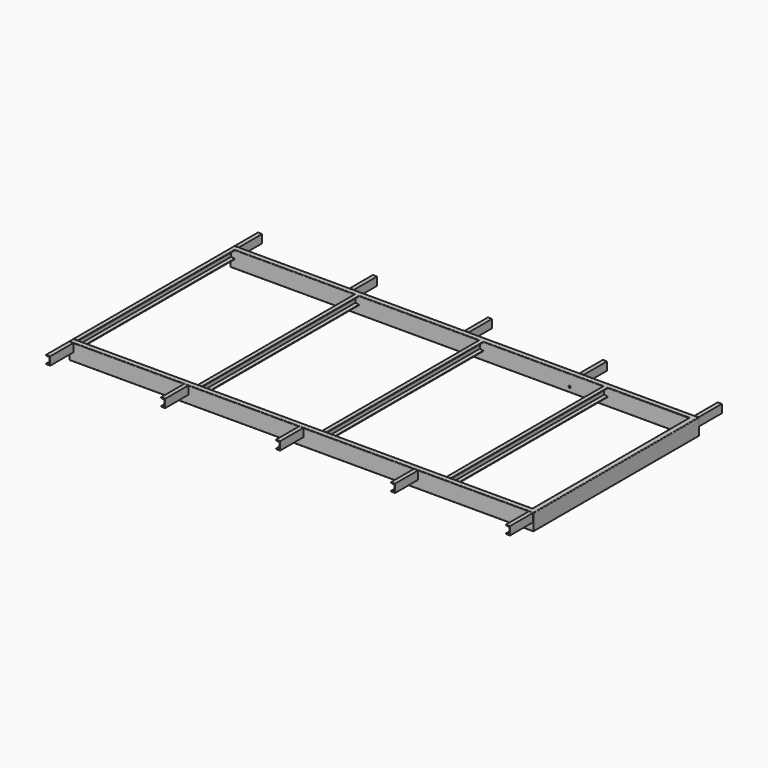
from build123d import *

# Parameters (mm, degrees)
F1_W      = 31.75
F1_H      = 133.35
F5_W      = 38.1
F5_H      = 5
F6_DEPTH  = 266.7
F7_W      = 38.1
F7_H      = 5
F8_DEPTH  = 266.7
F9_R      = 9.525
F10_DEPTH = 2640


with BuildPart() as f2:
    # F2: sweep along a path in F0
    with BuildLine(Plane.XY) as f2_path:
        Line((0, 0), (4221.5954545455, 0))
        Line((4221.5954545455, 0), (4221.5954545455, 1803.4))
        Line((4221.5954545455, 1803.4), (0, 1803.4))
    # F1 (on Right) → F2 (sweep)
    with BuildSketch(Plane.YZ):
        with BuildLine():
            ThreePointArc((0, -5), (-1.4644660941, -1.4644660941), (-5, 0))
            Line((-5, 0), (-45.8, 0))
            ThreePointArc((-45.8, 0), (-49.3355339059, -1.4644660941), (-50.8, -5))
            Line((-50.8, -5), (-50.8, -147.4))
            ThreePointArc((-50.8, -147.4), (-49.3355339059, -150.9355339059), (-45.8, -152.4))
            Line((-45.8, -152.4), (-5, -152.4))
            ThreePointArc((-5, -152.4), (-1.4644660941, -150.9355339059), (0, -147.4))
            Line((0, -147.4), (0, -5))
        make_face()
        with Locations((-25.4, -76.2)):
            Rectangle(F1_W, F1_H, mode=Mode.SUBTRACT)
    sweep(path=f2_path.line, transition=Transition.RIGHT)

    # F3 (on face) → F4 (join, up to the next surface of F2)
    with BuildSketch(Plane(origin=(0, 0, 0), x_dir=(-1, 0, 0), z_dir=(0, 1, 0))):
        Polygon((0, 0), (-38.1, 0), (-38.1, -5.08), (-6.35, -10), (-6.35, -66.2), (-38.1, -71.12), (-38.1, -76.2), (0, -76.2), align=None)
        Polygon((-1150.9375, -10), (-1150.9375, -66.2), (-1182.6875, -71.12), (-1182.6875, -76.2), (-1144.5875, -76.2), (-1144.5875, 0), (-1182.6875, 0), (-1182.6875, -5.08), align=None)
        Polygon((-2295.525, -10), (-2295.525, -66.2), (-2327.275, -71.12), (-2327.275, -76.2), (-2289.175, -76.2), (-2289.175, 0), (-2327.275, 0), (-2327.275, -5.08), align=None)
        Polygon((-3440.1125, -10), (-3440.1125, -66.2), (-3471.8625, -71.12), (-3471.8625, -76.2), (-3433.7625, -76.2), (-3433.7625, 0), (-3471.8625, 0), (-3471.8625, -5.08), align=None)
    extrude(until=Until.NEXT)

    # F5 (on face) → F6 (join)
    with BuildSketch(Plane.XZ.offset(50.8)):
        Polygon((38.1, -5), (0, -5), (0, -5.08), (31.75, -10), (31.75, -66.2), (0, -71.12), (0, -76.2), (38.1, -76.2), align=None)
        Polygon((1096.01, -5), (1057.91, -5), (1057.91, -5.08), (1089.66, -10), (1089.66, -66.2), (1057.91, -71.12), (1057.91, -76.2), (1096.01, -76.2), align=None)
        Polygon((2153.92, -5), (2115.82, -5), (2115.82, -5.08), (2147.57, -10), (2147.57, -66.2), (2115.82, -71.12), (2115.82, -76.2), (2153.92, -76.2), align=None)
        Polygon((3211.83, -5), (3173.73, -5), (3173.73, -5.08), (3205.48, -10), (3205.48, -66.2), (3173.73, -71.12), (3173.73, -76.2), (3211.83, -76.2), align=None)
        Polygon((4269.74, -76.2), (4269.74, -5), (4231.64, -5), (4231.64, -5.08), (4263.39, -10), (4263.39, -66.2), (4231.64, -71.12), (4231.64, -76.2), align=None)
        with Locations((4250.69, -2.5)):
            Rectangle(F5_W, F5_H)
        with Locations((3192.78, -2.5)):
            Rectangle(F5_W, F5_H)
        with Locations((2134.87, -2.5)):
            Rectangle(F5_W, F5_H)
        with Locations((1076.96, -2.5)):
            Rectangle(F5_W, F5_H)
        with Locations((19.05, -2.5)):
            Rectangle(F5_W, F5_H)
    extrude(amount=F6_DEPTH)

    # F7 (on face) → F8 (join)
    with BuildSketch(Plane(origin=(0, 1854.2, 0), x_dir=(-1, 0, 0), z_dir=(0, 1, 0))):
        Polygon((0, -5), (-38.1, -5), (-38.1, -76.2), (0, -76.2), (0, -71.12), (-31.75, -66.2), (-31.75, -10), (0, -5.08), align=None)
        with Locations((-19.05, -2.5)):
            Rectangle(F7_W, F7_H)
        with Locations((-1076.96, -2.5)):
            Rectangle(F7_W, F7_H)
        Polygon((-1057.91, -5.08), (-1057.91, -5), (-1096.01, -5), (-1096.01, -76.2), (-1057.91, -76.2), (-1057.91, -71.12), (-1089.66, -66.2), (-1089.66, -10), align=None)
        Polygon((-2115.82, -5.08), (-2115.82, -5), (-2153.92, -5), (-2153.92, -76.2), (-2115.82, -76.2), (-2115.82, -71.12), (-2147.57, -66.2), (-2147.57, -10), align=None)
        with Locations((-2134.87, -2.5)):
            Rectangle(F7_W, F7_H)
        with Locations((-3192.78, -2.5)):
            Rectangle(F7_W, F7_H)
        Polygon((-3173.73, -5.08), (-3173.73, -5), (-3211.83, -5), (-3211.83, -76.2), (-3173.73, -76.2), (-3173.73, -71.12), (-3205.48, -66.2), (-3205.48, -10), align=None)
        with Locations((-4250.69, -2.5)):
            Rectangle(F7_W, F7_H)
        Polygon((-4231.64, -5), (-4269.74, -5), (-4269.74, -76.2), (-4231.64, -76.2), (-4231.64, -71.12), (-4263.39, -66.2), (-4263.39, -10), (-4231.64, -5.08), align=None)
    extrude(amount=F8_DEPTH)

    # F9 (on face) → F10 (cut, symmetric)
    with BuildSketch(Plane.XZ.offset(-1803.4)):
        with Locations((3122.0374545455, -106.4)):
            Circle(F9_R)
    extrude(amount=F10_DEPTH, both=True, mode=Mode.SUBTRACT)


solid = f2.part
